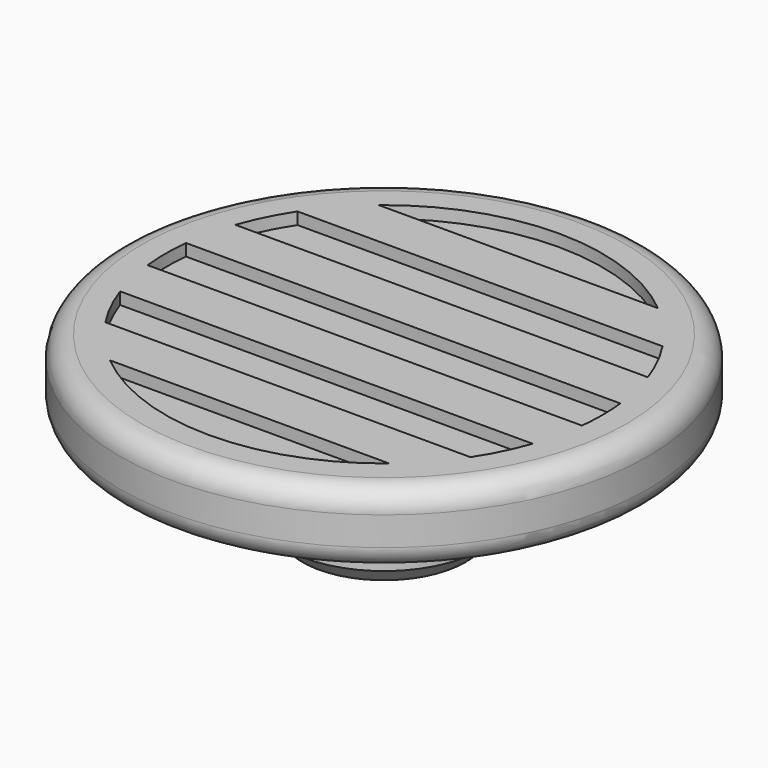
from build123d import *

# Parameters (mm, degrees)
F0_R     = 11
F0_R_2   = 5.5
F0_R_3   = 4.1
F1_DEPTH = 3
F2_DEPTH = 4.25
F3_SIZE  = 0.7
F4_R     = 0.9
F5_DEPTH = 0.5
F7_DEPTH = 0.5


with BuildPart() as f1:
    # F0 (on Top) → F1 (new body)
    with BuildSketch(Plane.XY):
        Circle(F0_R)
        Circle(F0_R_2, mode=Mode.SUBTRACT)
        Circle(F0_R_2)
        Circle(F0_R_3, mode=Mode.SUBTRACT)
        Circle(F0_R_3)
    extrude(amount=F1_DEPTH)

    # F0 (on Top) → F2 (join)
    with BuildSketch(Plane.XY):
        Circle(F0_R_3)
    extrude(amount=-F2_DEPTH)

    # F3
    f3_edges = [f1.edges().sort_by_distance(p)[0] for p in [
        (-4.1, 0, -4.25),
    ]]
    chamfer(f3_edges, length=F3_SIZE)

    # F4
    f4_edges = [f1.edges().sort_by_distance(p)[0] for p in [
        (11, 0, 1.5),
        (-11, 0, 0),
        (-11, 0, 3),
    ]]
    fillet(f4_edges, radius=F4_R)

    # F0 (on Top) → F5 (join)
    with BuildSketch(Plane.XY):
        Circle(F0_R_2)
        Circle(F0_R_3, mode=Mode.SUBTRACT)
    extrude(amount=-F5_DEPTH)

    # F6 (on face) → F7 (cut)
    with BuildSketch(Plane.XY.offset(3)):
        with BuildLine():
            ThreePointArc((1.3453624047, -9), (3.7170414054, -8.3062388113), (5.814636704, -7))
            Line((5.814636704, -7), (-5.814636704, -7))
            ThreePointArc((-5.814636704, -7), (-3.7170414054, -8.3062388113), (-1.3453624047, -9))
            Line((-1.3453624047, -9), (1.3453624047, -9))
        make_face()
        with BuildLine():
            ThreePointArc((7.6032887621, -5), (8.1587971524, -4.0303881979), (8.5912746435, -3))
            Line((8.5912746435, -3), (-8.5912746435, -3))
            ThreePointArc((-8.5912746435, -3), (-8.1587971524, -4.0303881979), (-7.6032887621, -5))
            Line((-7.6032887621, -5), (7.6032887621, -5))
        make_face()
        with BuildLine():
            ThreePointArc((9.044888059, -1), (9.0862115686, -0.5007587558), (9.1, 0))
            ThreePointArc((9.1, 0), (9.0862115686, 0.5007587558), (9.044888059, 1))
            Line((9.044888059, 1), (-9.044888059, 1))
            ThreePointArc((-9.044888059, 1), (-9.1, 0), (-9.044888059, -1))
            Line((-9.044888059, -1), (9.044888059, -1))
        make_face()
        with BuildLine():
            Line((-8.5912746435, 3), (8.5912746435, 3))
            ThreePointArc((8.5912746435, 3), (8.1587971524, 4.0303881979), (7.6032887621, 5))
            Line((7.6032887621, 5), (-7.6032887621, 5))
            ThreePointArc((-7.6032887621, 5), (-8.1587971524, 4.0303881979), (-8.5912746435, 3))
        make_face()
        with BuildLine():
            Line((-5.814636704, 7), (5.814636704, 7))
            ThreePointArc((5.814636704, 7), (3.7170414054, 8.3062388113), (1.3453624047, 9))
            Line((1.3453624047, 9), (-1.3453624047, 9))
            ThreePointArc((-1.3453624047, 9), (-3.7170414054, 8.3062388113), (-5.814636704, 7))
        make_face()
        with BuildLine():
            ThreePointArc((-1.3453624047, -9), (0, -9.1), (1.3453624047, -9))
            Line((1.3453624047, -9), (-1.3453624047, -9))
        make_face()
        with BuildLine():
            Line((-1.3453624047, 9), (1.3453624047, 9))
            ThreePointArc((1.3453624047, 9), (0, 9.1), (-1.3453624047, 9))
        make_face()
    extrude(amount=-F7_DEPTH, mode=Mode.SUBTRACT)


solid = f1.part
